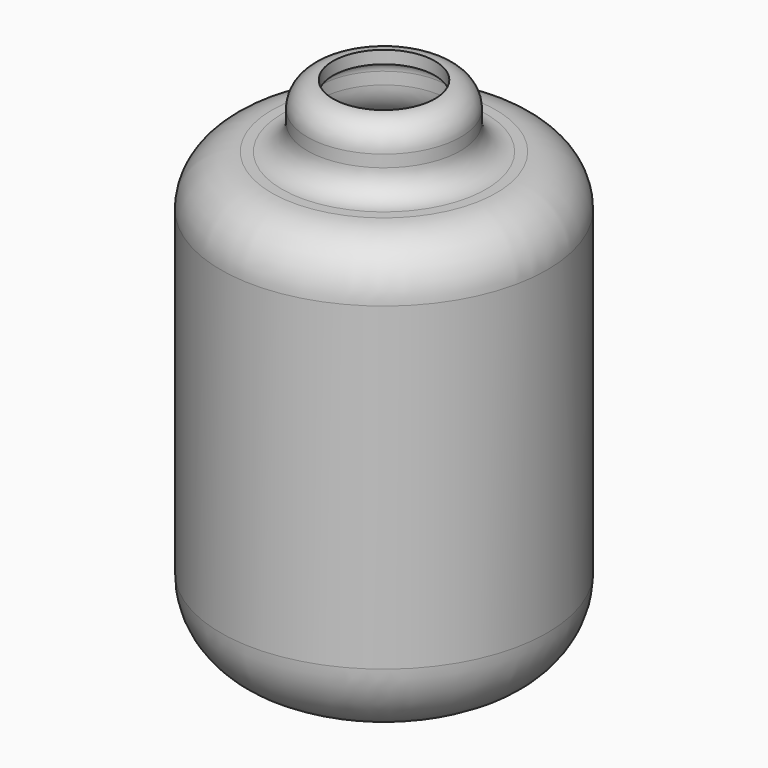
from build123d import *

# Parameters (mm, degrees)
F2_T = -2.5


# Not quite as in the source:
# - a shell that OpenCascade refuses in one call is made with other operations: the cavity is built on its own and cut out


with BuildPart() as f1:
    # F0 (on Front) → F1 (revolve)
    with BuildSketch(Plane.XZ):
        with BuildLine():
            Line((0, -50), (0, 50))
            Line((0, 50), (-10, 50))
            ThreePointArc((-10, 50), (-13.5355339059, 48.5355339059), (-15, 45))
            Line((-15, 45), (-15, 42.6380823553))
            ThreePointArc((-15, 42.6380823553), (-16.4644660941, 39.1025484493), (-20, 37.6380823553))
            Line((-20, 37.6380823553), (-22, 37.6380823553))
            ThreePointArc((-22, 37.6380823553), (-29.0710678119, 34.7091501671), (-32, 27.6380823553))
            Line((-32, 27.6380823553), (-32, -35))
            ThreePointArc((-32, -35), (-27.6066017178, -45.6066017178), (-17, -50))
            Line((-17, -50), (0, -50))
        make_face()
    revolve(axis=Axis((0, 0, 0), (0, 0, -1)))

    # F2: a shell. OpenCascade refuses it in one call, so the cavity is built on its own and cut out:
    # the body offset inwards by the wall thickness, plus a prism from it out through each open face.
    f2_core = offset(f1.part, amount=F2_T, mode=Mode.PRIVATE)
    f2_exits = [f2_core.faces().sort_by_distance(p)[0] for p in [
        (0, 0, 47.5),
    ]]
    add(f2_core, mode=Mode.SUBTRACT)
    extrude(f2_exits, amount=-F2_T, mode=Mode.SUBTRACT)


solid = f1.part
